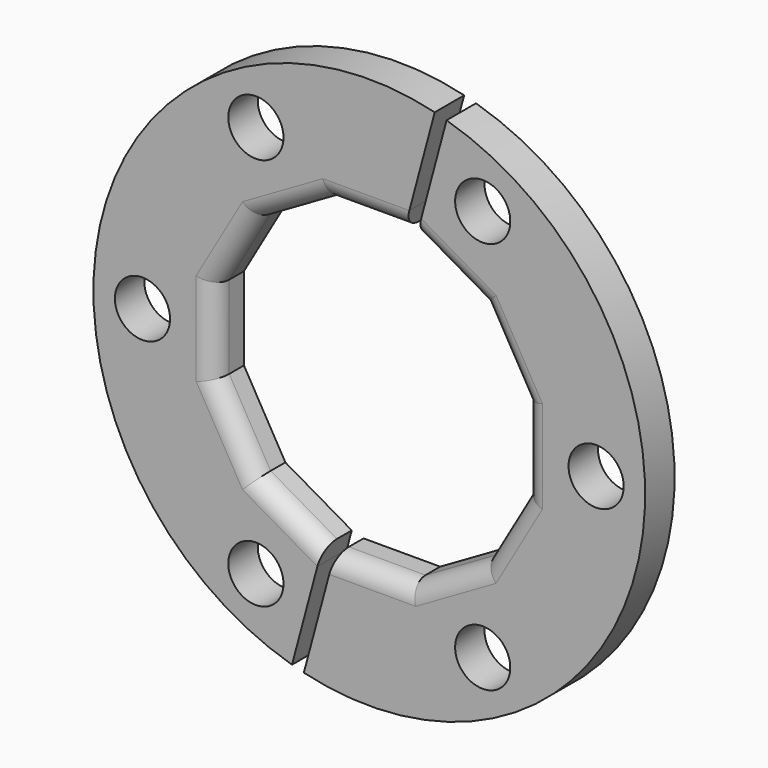
from build123d import *

# Parameters (mm, degrees)
F0_R            = 45
F1_DEPTH        = 3
F2_R            = 3
F3_R            = 4.5
F4_DEPTH        = 12.5
F4_COPIES_COUNT = 6
F6_DEPTH        = 25


# Not quite as in the source:
# - a pattern or mirror of a feature is missing from the dataset's text; its kind, count and spacing are read off the source's solid


with BuildPart() as f1:
    # F0 (on Front) → F1 (new body, symmetric)
    with BuildSketch(Plane.XZ):
        Circle(F0_R)
        Polygon((-18.4842828911, 18.4842828911), (-6.7657171089, 25.25), (6.7657171089, 25.25), (18.4842828911, 18.4842828911), (25.25, 6.7657171089), (25.25, -6.7657171089), (18.4842828911, -18.4842828911), (6.7657171089, -25.25), (-6.7657171089, -25.25), (-18.4842828911, -18.4842828911), (-25.25, -6.7657171089), (-25.25, 6.7657171089), align=None, mode=Mode.SUBTRACT)
    extrude(amount=F1_DEPTH, both=True)

    # F2
    f2_edges = [f1.edges().sort_by_distance(p)[0] for p in [
        (-12.625, -3, 21.867141),
        (0, -3, 25.25),
        (12.625, -3, 21.867141),
        (21.867141, -3, 12.625),
        (25.25, -3, 0),
        (21.867141, -3, -12.625),
        (12.625, -3, -21.867141),
        (0, -3, -25.25),
        (-12.625, -3, -21.867141),
        (-21.867141, -3, -12.625),
        (-25.25, -3, 0),
        (-21.867141, -3, 12.625),
    ]]
    fillet(f2_edges, radius=F2_R)

    # F3 (on Front) → F4 (cut, symmetric)
    with BuildSketch(Plane.XZ):
        with Locations((37, 0)):
            Circle(F3_R)
    f4 = extrude(amount=F4_DEPTH, both=True, mode=Mode.SUBTRACT)

    # F4_copies: F4 ×6 about axis
    f4_copies_axis = Axis((0, 0, 0), (0, 1, 0))
    for i in range(1, F4_COPIES_COUNT):
        add(f4.rotate(f4_copies_axis, i * 360 / F4_COPIES_COUNT), mode=Mode.SUBTRACT)

    # F5 (on face) → F6 (cut)
    with BuildSketch(Plane.XZ.offset(3)):
        with BuildLine():
            Line((-8.4661401583, -27.7323619098), (-12.6099067336, -43.1971093034))
            ThreePointArc((-12.6099067336, -43.1971093034), (-11.6468570296, -43.466662183), (-10.678055081, -43.7147473936))
            Line((-10.678055081, -43.7147473936), (-6.5342885058, -28.25))
            Line((-6.5342885058, -28.25), (-7.5695646862, -28.25))
            Line((-7.5695646862, -28.25), (-8.4661401583, -27.7323619098))
        make_face()
        with BuildLine():
            ThreePointArc((12.6099067336, 43.1971093034), (11.6468570296, 43.466662183), (10.678055081, 43.7147473936))
            Line((10.678055081, 43.7147473936), (6.5342885058, 28.25))
            Line((6.5342885058, 28.25), (7.5695646862, 28.25))
            Line((7.5695646862, 28.25), (8.4661401583, 27.7323619098))
            Line((8.4661401583, 27.7323619098), (12.6099067336, 43.1971093034))
        make_face()
        Polygon((6.5342885058, 28.25), (-8.4661401583, -27.7323619098), (-7.5695646862, -28.25), (-6.5342885058, -28.25), (8.4661401583, 27.7323619098), (7.5695646862, 28.25), align=None)
    extrude(amount=-F6_DEPTH, mode=Mode.SUBTRACT)


solid = f1.part
